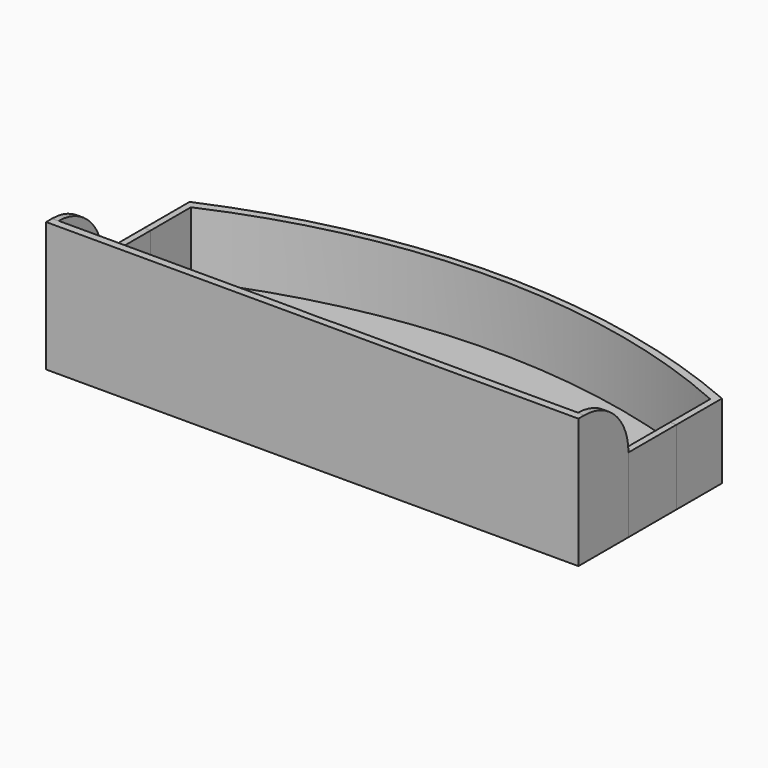
from build123d import *

# Parameters (mm, degrees)
F1_DEPTH    = 3
F2_DEPTH    = 40
F3_DEPTH    = 23
F4_DEPTH    = 23
F5_T1_DEPTH = 87
F6_T1_DEPTH = 87
F7_DEPTH    = 23
F8_DEPTH    = 23


# Not quite as in the source:
# - a fillet or chamfer that OpenCascade refuses, or shapes differently, is made with other operations: its cross-section is extruded or revolved along the edge and cut away or added


with BuildPart() as f1:
    # F0 (on Top) → F1 (new body)
    with BuildSketch(Plane.XY):
        with BuildLine():
            Line((-58.0038166074, 15.5), (-58.0038166074, 0))
            Line((-58.0038166074, 0), (-58.0038166074, -3))
            Line((-58.0038166074, -3), (-58.0038166074, -18.5))
            ThreePointArc((-58.0038166074, -18.5), (-22.0977805804, -30.4949807288), (15.4409240709, -35.3907583952))
            Line((15.4409240709, -35.3907583952), (28.5514427142, -35.3907583952))
            ThreePointArc((28.5514427142, -35.3907583952), (66.0901473656, -30.4949807288), (101.9961833926, -18.5))
            Line((101.9961833926, -18.5), (101.9961833926, -15.5))
            Line((101.9961833926, -15.5), (101.9961833926, -3))
            Line((101.9961833926, -3), (101.9961833926, 0))
            Line((101.9961833926, 0), (101.9961833926, 15.5))
            ThreePointArc((101.9961833926, 15.5), (21.9961833926, 32.5), (-58.0038166074, 15.5))
        make_face()
    extrude(amount=F1_DEPTH)

    # F0 (on Top) → F2 (join)
    with BuildSketch(Plane.XY):
        with BuildLine():
            Line((-58.0038166074, -35.3907583952), (-58.0038166074, -18.5))
            Line((-58.0038166074, -18.5), (-60.0038166074, -18.5))
            Line((-60.0038166074, -18.5), (-60.0038166074, -20.5))
            Line((-60.0038166074, -20.5), (-60.0038166074, -37.7693227232))
            Line((-60.0038166074, -37.7693227232), (103.9961833926, -37.7693227232))
            Line((103.9961833926, -37.7693227232), (103.9961833926, -20.5))
            Line((103.9961833926, -20.5), (103.9961833926, -18.5))
            Line((103.9961833926, -18.5), (101.9961833926, -18.5))
            Line((101.9961833926, -18.5), (101.9961833926, -35.3907583952))
            Line((101.9961833926, -35.3907583952), (28.5514427142, -35.3907583952))
            ThreePointArc((28.5514427142, -35.3907583952), (21.9961833926, -35.5), (15.4409240709, -35.3907583952))
            Line((15.4409240709, -35.3907583952), (-58.0038166074, -35.3907583952))
        make_face()
    extrude(amount=F2_DEPTH)

    # F5: fillet of radius 17 on 1 edges, made by hand

    # F5_s2 → F5_t1 (cut)
    with BuildSketch(Plane.YZ.offset(-102.5038166074)):
        with BuildLine():
            ThreePointArc((-35.5, 40), (-23.4791847198, 35.0208152802), (-18.5, 23))
            Line((-18.5, 23), (-18.5, 40))
            Line((-18.5, 40), (-35.5, 40))
        make_face()
    extrude(amount=F5_T1_DEPTH, mode=Mode.SUBTRACT)

    # F6: fillet of radius 17 on 1 edges, made by hand

    # F6_s2 → F6_t1 (cut)
    with BuildSketch(Plane.YZ.offset(59.4961833926)):
        with BuildLine():
            ThreePointArc((-18.5, 23), (-23.4791847198, 35.0208152802), (-35.5, 40))
            Line((-35.5, 40), (-18.5, 40))
            Line((-18.5, 40), (-18.5, 23))
        make_face()
    extrude(amount=F6_T1_DEPTH, mode=Mode.SUBTRACT)


with BuildPart() as f3:
    # F0 (on Top) → F3 (new body)
    with BuildSketch(Plane.XY):
        with BuildLine():
            Line((-60.0038166074, 0), (-58.0038166074, 0))
            Line((-58.0038166074, 0), (-58.0038166074, 15.5))
            ThreePointArc((-58.0038166074, 15.5), (21.9961833926, 32.5), (101.9961833926, 15.5))
            Line((101.9961833926, 15.5), (101.9961833926, 0))
            Line((101.9961833926, 0), (103.9961833926, 0))
            Line((103.9961833926, 0), (103.9961833926, 17.5))
            ThreePointArc((103.9961833926, 17.5), (21.9961833926, 34.5), (-60.0038166074, 17.5))
            Line((-60.0038166074, 17.5), (-60.0038166074, 0))
        make_face()
    extrude(amount=F3_DEPTH)


with BuildPart() as f4:
    # F0 (on Top) → F4 (new body)
    with BuildSketch(Plane.XY):
        with BuildLine():
            ThreePointArc((101.9961833926, -18.5), (66.0901473656, -30.4949807288), (28.5514427142, -35.3907583952))
            Line((28.5514427142, -35.3907583952), (101.9961833926, -35.3907583952))
            Line((101.9961833926, -35.3907583952), (101.9961833926, -18.5))
        make_face()
    extrude(amount=F4_DEPTH)


with BuildPart() as f4b:
    # F0 (on Top) → F4, piece 2 (new body)
    with BuildSketch(Plane.XY):
        with BuildLine():
            ThreePointArc((15.4409240709, -35.3907583952), (-22.0977805804, -30.4949807288), (-58.0038166074, -18.5))
            Line((-58.0038166074, -18.5), (-58.0038166074, -35.3907583952))
            Line((-58.0038166074, -35.3907583952), (15.4409240709, -35.3907583952))
        make_face()
    extrude(amount=F4_DEPTH)


with BuildPart() as f7:
    # F0 (on Top) → F7 (new body)
    with BuildSketch(Plane.XY):
        Polygon((-58.0038166074, -3), (-58.0038166074, 0), (-60.0038166074, 0), (-60.0038166074, -3), (-60.0038166074, -18.5), (-58.0038166074, -18.5), align=None)
    extrude(amount=F7_DEPTH)


with BuildPart() as f8:
    # F0 (on Top) → F8 (new body)
    with BuildSketch(Plane.XY):
        Polygon((103.9961833926, 0), (101.9961833926, 0), (101.9961833926, -3), (101.9961833926, -15.5), (101.9961833926, -18.5), (103.9961833926, -18.5), (103.9961833926, -17.5), (103.9961833926, -3), align=None)
    extrude(amount=F8_DEPTH)


solid = Compound([f1.part, f3.part, f4.part, f4b.part, f7.part, f8.part])
